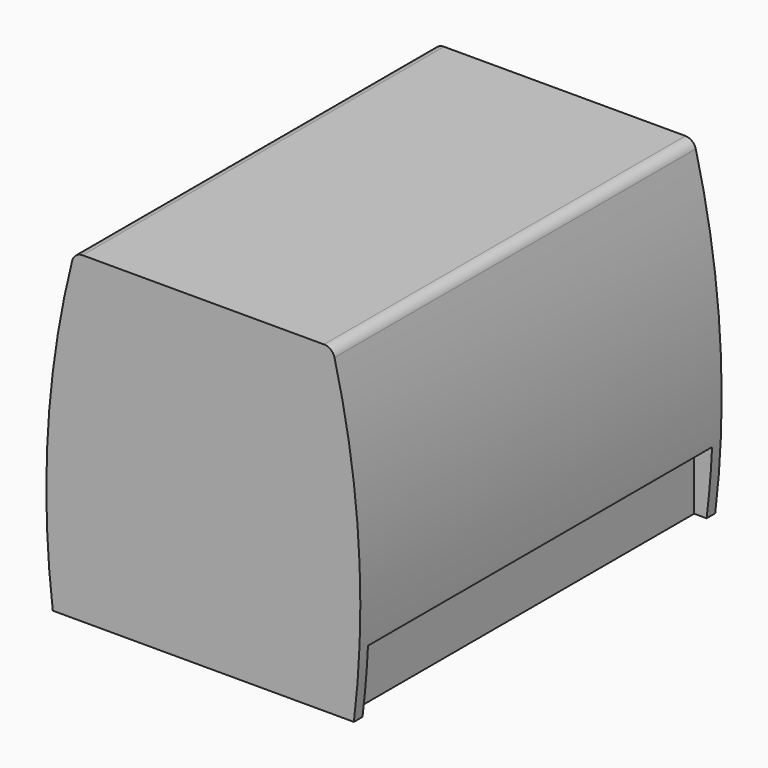
from build123d import *

# Parameters (mm, degrees)
F1_DEPTH = 1050
F2_W     = 200
F2_H     = 300
F3_DEPTH = 1000
F4_R     = 50


# Not quite as in the source:
# - a pattern or mirror of a feature is missing from the dataset's text; its kind, count and spacing are read off the source's solid


with BuildPart() as f1:
    # F0 (on Front) → F1 (new body, symmetric)
    with BuildSketch(Plane.XZ):
        with BuildLine():
            ThreePointArc((-600, 1500), (-721.1019148035, 754.7401276536), (-700, 0))
            Line((-700, 0), (700, 0))
            ThreePointArc((700, 0), (721.1019148035, 754.7401276536), (600, 1500))
            Line((600, 1500), (-600, 1500))
        make_face()
    extrude(amount=F1_DEPTH, both=True)

    # F2 (on Front) → F3 (cut, symmetric)
    with BuildSketch(Plane.XZ):
        with Locations((-742.0543789864, 150)):
            Rectangle(F2_W, F2_H)
    f3 = extrude(amount=F3_DEPTH, both=True, mode=Mode.SUBTRACT)

    # F3_copies: F3 across plane
    add(f3.mirror(Plane(origin=(0, 0, 0), x_dir=(0, 0, 1), z_dir=(1, 0, 0))), mode=Mode.SUBTRACT)

    # F4
    f4_edges = [f1.edges().sort_by_distance(p)[0] for p in [
        (600, 0, 1500),
        (-600, 0, 1500),
    ]]
    fillet(f4_edges, radius=F4_R)


solid = f1.part
